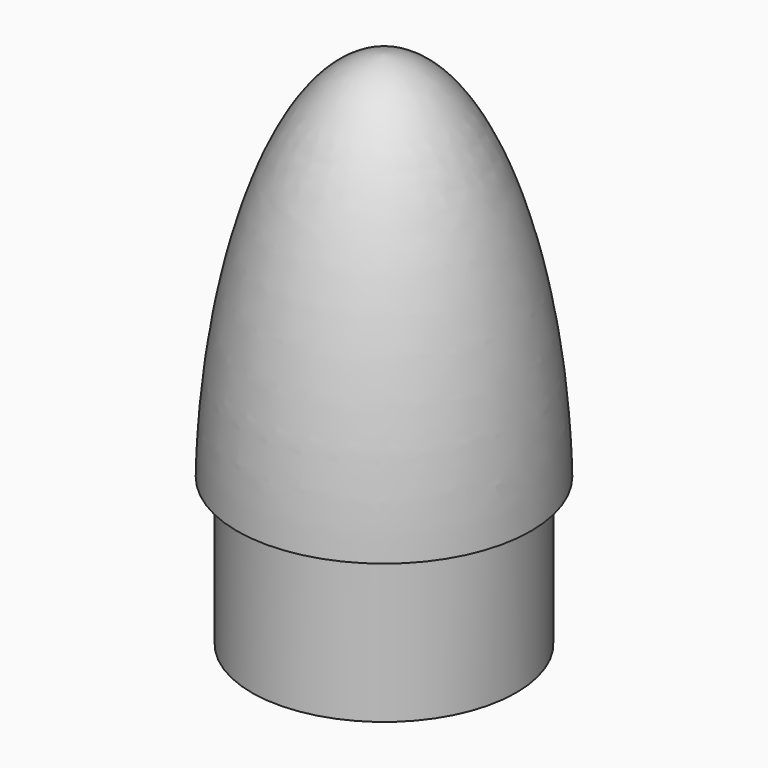
from build123d import *

# Parameters (mm, degrees)
F4_D     = 3
F4_DEPTH = 12
F4_TIP   = 0.9012909285


with BuildPart() as f1:
    # F0 (on Front) → F1 (revolve)
    with BuildSketch(Plane.XZ):
        with BuildLine():
            add(Edge.make_bspline(
                [(26.8895727958, 3), (26.9346478476, 2.0004075938), (26.9715210375, 1.0001471851), (27, 0)],
                knots=[74.7734725715, 74.7734725715, 74.7734725715, 74.7734725715, 76.8960337079, 76.8960337079, 76.8960337079, 76.8960337079], degree=3))
            Line((27, 0), (30, 0))
            add(Edge.make_bspline(
                [(0, 76), (18.2135365903, 75.0966593623), (29.3766844422, 35.9996296465), (30, 0)],
                knots=[0, 0, 0, 0, 81.7067928633, 81.7067928633, 81.7067928633, 81.7067928633], degree=3))
            Line((0, 76), (0, 72))
            add(Edge.make_bspline(
                [(0, 72), (13.535191017, 72.5981812348), (25.3016712319, 38.2135889442), (26.8895727958, 3)],
                knots=[0, 0, 0, 0, 74.7734725715, 74.7734725715, 74.7734725715, 74.7734725715], degree=3))
        make_face()
        with BuildLine():
            Line((27, -30), (27, 0))
            add(Edge.make_bspline(
                [(26.8895727958, 3), (26.9346478476, 2.0004075938), (26.9715210375, 1.0001471851), (27, 0)],
                knots=[74.7734725715, 74.7734725715, 74.7734725715, 74.7734725715, 76.8960337079, 76.8960337079, 76.8960337079, 76.8960337079], degree=3))
            Line((26.8895727958, 3), (24, 3))
            Line((24, 3), (24, 0))
            Line((24, 0), (24, -25))
            Line((24, -25), (0, -25))
            Line((0, -25), (0, -30))
            Line((0, -30), (27, -30))
        make_face()
    revolve(axis=Axis((0, 0, 36), (0, 0, 1)))

    # F4
    with Locations(Plane(origin=(0, 0, -30), x_dir=(1, 0, 0), z_dir=(0, 0, -1))):
        with Locations((0, 0)):
            Hole(F4_D / 2, depth=F4_DEPTH)
            with Locations((0, 0, -(F4_DEPTH + F4_TIP / 2))):  # 118° drill point
                Cone(0, F4_D / 2, F4_TIP, mode=Mode.SUBTRACT)


solid = f1.part
